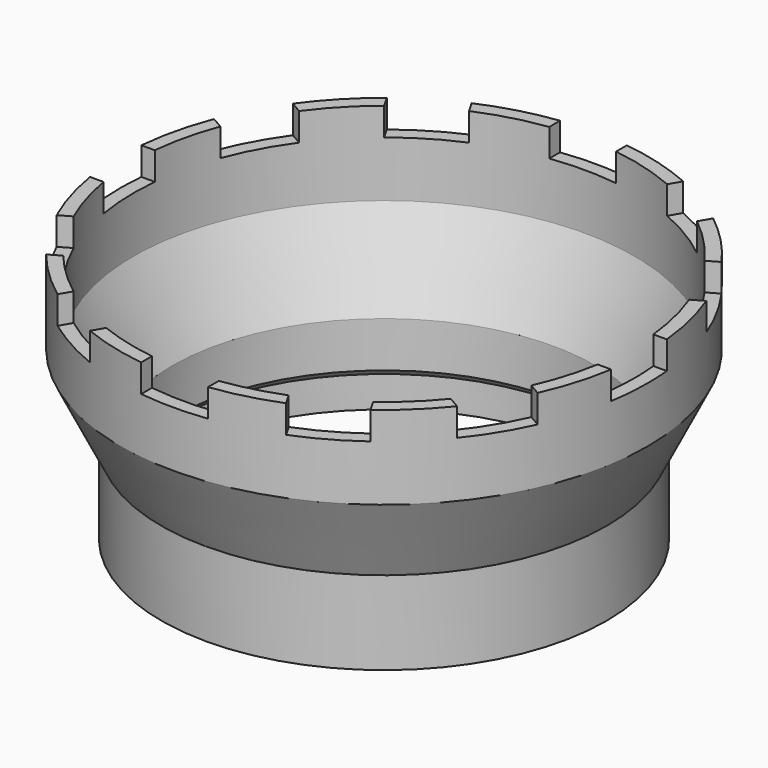
from build123d import *

# Parameters (mm, degrees)
F0_R     = 40
F0_R_2   = 38
F1_DEPTH = 15
F2_W     = 2
F2_H     = 5.6
F5_W     = 12
F5_H     = 12
F6_DEPTH = 5
F7_SIZE  = 1.19999


# Not quite as in the source:
# - a fillet or chamfer is up to 0.001 mm smaller than in the source, because OpenCascade refuses the exact size


with BuildPart() as f1:
    # F0 (on Top) → F1 (new body)
    with BuildSketch(Plane.XY):
        Circle(F0_R)
        Circle(F0_R_2, mode=Mode.SUBTRACT)
    extrude(amount=F1_DEPTH)

    # F2 (on Front) → F3 (revolve, cut)
    with BuildSketch(Plane.XZ):
        with Locations((38.2, 2.8)):
            Rectangle(F2_W, F2_H)
        Polygon((45, 30), (38, 15), (40, 15), (47.4, 30), (47.4, 45), (45, 45), align=None)
    revolve(axis=Axis((0, 0, 15), (0, 0, 1)), mode=Mode.SUBTRACT)

    # F2 (on Front) → F4 (revolve)
    with BuildSketch(Plane.XZ):
        Polygon((45, 30), (38, 15), (40, 15), (47.4, 30), (47.4, 45), (45, 45), align=None)
    revolve(axis=Axis((0, 0, 15), (0, 0, 1)))

    # F5 (on face) → F6 (cut)
    with BuildSketch(Plane.XY.offset(45)):
        with Locations((0, 46)):
            Rectangle(F5_W, F5_H)
        Polygon((-15.5538475773, 37.4400542571), (-21.5538475773, 47.8323591025), (-31.9461524227, 41.8323591025), (-25.9461524227, 31.4400542571), align=None)
        Polygon((-32.9400542571, 24.4461524227), (-43.3323591025, 30.4461524227), (-49.3323591025, 20.0538475773), (-38.9400542571, 14.0538475773), align=None)
        with Locations((-47.5, -1.5)):
            Rectangle(F5_W, F5_H)
        Polygon((-38.9400542571, -17.0538475773), (-49.3323591025, -23.0538475773), (-43.3323591025, -33.4461524227), (-32.9400542571, -27.4461524227), align=None)
        Polygon((-25.9461524227, -34.4400542571), (-31.9461524227, -44.8323591025), (-21.5538475773, -50.8323591025), (-15.5538475773, -40.4400542571), align=None)
        with Locations((0, -49)):
            Rectangle(F5_W, F5_H)
        Polygon((15.5538475773, -40.4400542571), (21.5538475773, -50.8323591025), (31.9461524227, -44.8323591025), (25.9461524227, -34.4400542571), align=None)
        Polygon((32.9400542571, -27.4461524227), (43.3323591025, -33.4461524227), (49.3323591025, -23.0538475773), (38.9400542571, -17.0538475773), align=None)
        with Locations((47.5, -1.5)):
            Rectangle(F5_W, F5_H)
        Polygon((38.9400542571, 14.0538475773), (49.3323591025, 20.0538475773), (43.3323591025, 30.4461524227), (32.9400542571, 24.4461524227), align=None)
        Polygon((25.9461524227, 31.4400542571), (31.9461524227, 41.8323591025), (21.5538475773, 47.8323591025), (15.5538475773, 37.4400542571), align=None)
    extrude(amount=-F6_DEPTH, mode=Mode.SUBTRACT)

    # F7 (size 1.2 in the source; OpenCascade refuses exactly that, so slightly less here)
    f7_edges = [f1.edges().sort_by_distance(p)[0] for p in [
        (-38, 0, 5.6),
    ]]
    chamfer(f7_edges, length=F7_SIZE)


solid = f1.part
